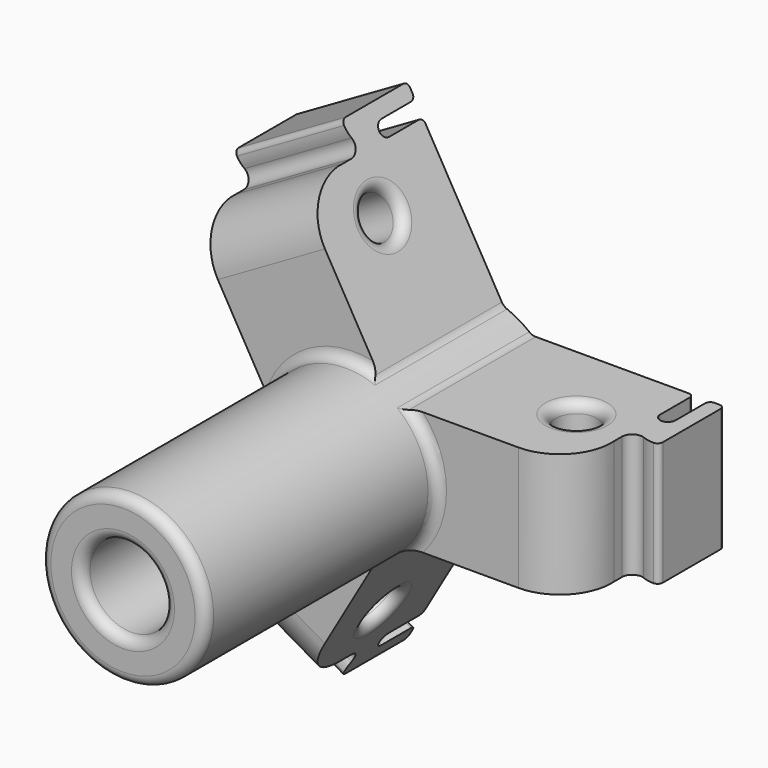
from build123d import *

# Parameters (mm, degrees)
F0_R          = 8
F0_R_2        = 4
F1_DEPTH      = 35
F1_DEPTH_BACK = 8
F2_R          = 2
F3_DEPTH      = 6
F4_R          = 1
F5_COUNT      = 3


# Not quite as in the source:
# - a feature of the source that left no trace in its solid (it failed there, or was rolled back) is left out
# - a feature names something its author has since deleted; it is built from what else it names


with BuildPart() as f1:
    # F0 (on Front) → F1 (new body, two sides)
    with BuildSketch(Plane.XZ) as f1_sk:
        with Locations((-66, 0)):
            Circle(F0_R)
        with Locations((-66, 0)):
            Circle(F0_R_2, mode=Mode.SUBTRACT)
    extrude(amount=F1_DEPTH)
    extrude(f1_sk.sketch, amount=-F1_DEPTH_BACK)

    # F2 (on Top) → F3 (join, symmetric)
    with BuildSketch(Plane.XY):
        with BuildLine():
            Line((-45.5077314954, 8), (-62, 8))
            Line((-62, 8), (-62, -7))
            Line((-62, -7), (-50, -7))
            ThreePointArc((-50, -7), (-46.3485162833, -5.4156502553), (-45.0111234843, -1.6666666667))
            Line((-45.0111234843, -1.6666666667), (-45.0111234843, 1.3333333333))
            ThreePointArc((-45.0111234843, 1.3333333333), (-43.9308987888, 0.3542486889), (-42.5166852265, 0))
            ThreePointArc((-42.5166852265, 0), (-42.1631318359, 0.1464466094), (-42.0166852265, 0.5))
            Line((-42.0166852265, 0.5), (-42.0166852265, 7.5))
            ThreePointArc((-42.0166852265, 7.5), (-42.1631318359, 7.8535533906), (-42.5166852265, 8))
            Line((-42.5166852265, 8), (-43.0077314954, 8))
            ThreePointArc((-43.0077314954, 8), (-43.361284886, 7.8535533906), (-43.5077314954, 7.5))
            Line((-43.5077314954, 7.5), (-43.5077314954, 3.9235844234))
            ThreePointArc((-43.5077314954, 3.9235844234), (-44.2577314954, 3.1735844234), (-45.0077314954, 3.9235844234))
            Line((-45.0077314954, 3.9235844234), (-45.0077314954, 7.5))
            ThreePointArc((-45.0077314954, 7.5), (-45.1541781048, 7.8535533906), (-45.5077314954, 8))
        make_face()
        with Locations((-50, 0)):
            Circle(F2_R, mode=Mode.SUBTRACT)
    extrude(amount=F3_DEPTH, both=True)

    # F4
    f4_edges = [f1.edges().sort_by_distance(p)[0] for p in [
        (-52, 0, 6),
        (-52, 0, -6),
        (-70, 8, 0),
        (-70, -35, 0),
        (-74, -35, 0),
        (-58.708497, -7, 3.291503),
        (-60.708497, -3.5, 6),
        (-60.708497, -3.5, -6),
        (-58.708497, -7, -3.291503),
        (-45.011123, 1.333333, 0),
        (-60.708497, 4, -6),
        (-60.708497, 4, 6),
    ]]
    fillet(f4_edges, radius=F4_R)

    # F5: F1 ×3 about axis
    f5_axis = Axis((-66, -34, 0), (0, -1, 0))


with BuildPart() as f1_1:
    add(f1.part)
    for i in range(1, F5_COUNT):
        add(f1.part.rotate(f5_axis, i * 360 / F5_COUNT))


solid = f1_1.part
